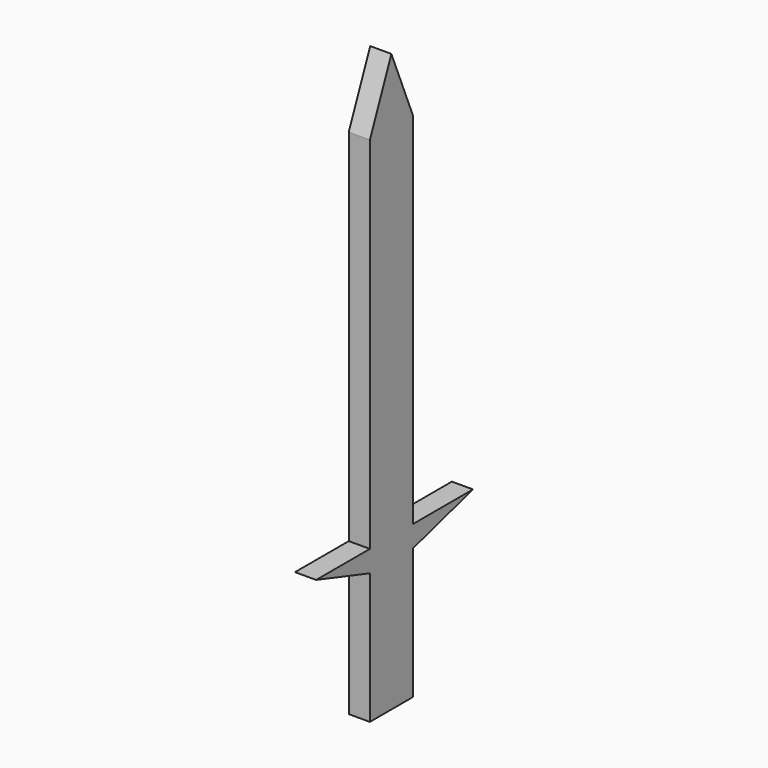
from build123d import *

# Parameters (mm, degrees)
F1_DEPTH    = 2.54
F2_T1_DEPTH = 28.6682991577
F3_DEPTH    = 2.54
F4_DEPTH    = 2.54
F5_T1_DEPTH = 28.6682991577
F6_T1_DEPTH = 28.8815311919


# Not quite as in the source:
# - a fillet or chamfer that OpenCascade refuses, or shapes differently, is made with other operations: its cross-section is extruded or revolved along the edge and cut away or added


with BuildPart() as f1:
    # F0 (on Right) → F1 (new body)
    with BuildSketch(Plane.YZ):
        Polygon((-57.2273433208, -53.503472358), (-49.1374544799, -56.0896545649), (-49.1374544799, -53.503472358), align=None)
        Polygon((-49.1374544799, -53.503472358), (-49.1374544799, -56.0896545649), (-42.6720008254, -56.0896545649), (-42.6720008254, -53.503472358), (-42.6720008254, 0), (-49.1374544799, 0), align=None)
        with BuildLine():
            Line((-42.6720008254, -56.0896545649), (-49.1374544799, -56.0896545649))
            Line((-49.1374544799, -56.0896545649), (-49.1374544799, -67.4042031169))
            ThreePointArc((-49.1374544799, -67.4042031169), (-45.9047276527, -64.1714762896), (-42.6720008254, -67.4042031169))
            Line((-42.6720008254, -67.4042031169), (-42.6720008254, -56.0896545649))
        make_face()
        Polygon((-42.6720008254, -53.503472358), (-42.6720008254, -56.0896545649), (-33.620364964, -53.503472358), align=None)
        with BuildLine():
            ThreePointArc((-42.6720008254, -67.4042031169), (-45.9047276527, -70.6369299442), (-49.1374544799, -67.4042031169))
            Line((-49.1374544799, -67.4042031169), (-49.1374544799, -71.8398466706))
            Line((-49.1374544799, -71.8398466706), (-42.6720008254, -71.8398466706))
            Line((-42.6720008254, -71.8398466706), (-42.6720008254, -67.4042031169))
        make_face()
        with BuildLine():
            ThreePointArc((-42.6720008254, -67.4042031169), (-45.9047276527, -64.1714762896), (-49.1374544799, -67.4042031169))
            ThreePointArc((-49.1374544799, -67.4042031169), (-45.9047276527, -70.6369299442), (-42.6720008254, -67.4042031169))
        make_face()
    extrude(amount=F1_DEPTH)

    # F2: chamfer of 5.08 on 2 edges, made by hand

    # F2_s2 → F2_t1 (cut)
    with BuildSketch(Plane.YZ.offset(-13.0641495789)):
        Polygon((-44.0574544799, 0), (-49.1374544799, -5.08), (-49.1374544799, 0), align=None)
        Polygon((-42.6720008254, -5.08), (-47.7520008254, 0), (-42.6720008254, 0), align=None)
    extrude(amount=F2_T1_DEPTH, mode=Mode.SUBTRACT)

    # F0 (on Right) → F3 (join)
    with BuildSketch(Plane.YZ):
        Polygon((-57.2273433208, -53.503472358), (-49.1374544799, -56.0896545649), (-49.1374544799, -53.503472358), align=None)
        Polygon((-49.1374544799, -53.503472358), (-49.1374544799, -56.0896545649), (-42.6720008254, -56.0896545649), (-42.6720008254, -53.503472358), (-42.6720008254, 0), (-49.1374544799, 0), align=None)
        with BuildLine():
            Line((-42.6720008254, -56.0896545649), (-49.1374544799, -56.0896545649))
            Line((-49.1374544799, -56.0896545649), (-49.1374544799, -67.4042031169))
            ThreePointArc((-49.1374544799, -67.4042031169), (-45.9047276527, -64.1714762896), (-42.6720008254, -67.4042031169))
            Line((-42.6720008254, -67.4042031169), (-42.6720008254, -56.0896545649))
        make_face()
        Polygon((-42.6720008254, -53.503472358), (-42.6720008254, -56.0896545649), (-33.620364964, -53.503472358), align=None)
        with BuildLine():
            ThreePointArc((-42.6720008254, -67.4042031169), (-45.9047276527, -70.6369299442), (-49.1374544799, -67.4042031169))
            Line((-49.1374544799, -67.4042031169), (-49.1374544799, -71.8398466706))
            Line((-49.1374544799, -71.8398466706), (-42.6720008254, -71.8398466706))
            Line((-42.6720008254, -71.8398466706), (-42.6720008254, -67.4042031169))
        make_face()
        with BuildLine():
            ThreePointArc((-42.6720008254, -67.4042031169), (-45.9047276527, -64.1714762896), (-49.1374544799, -67.4042031169))
            ThreePointArc((-49.1374544799, -67.4042031169), (-45.9047276527, -70.6369299442), (-42.6720008254, -67.4042031169))
        make_face()
    extrude(amount=F3_DEPTH)

    # F0 (on Right) → F4 (join)
    with BuildSketch(Plane.YZ):
        Polygon((-57.2273433208, -53.503472358), (-49.1374544799, -56.0896545649), (-49.1374544799, -53.503472358), align=None)
        Polygon((-49.1374544799, -53.503472358), (-49.1374544799, -56.0896545649), (-42.6720008254, -56.0896545649), (-42.6720008254, -53.503472358), (-42.6720008254, 0), (-49.1374544799, 0), align=None)
        with BuildLine():
            Line((-42.6720008254, -56.0896545649), (-49.1374544799, -56.0896545649))
            Line((-49.1374544799, -56.0896545649), (-49.1374544799, -67.4042031169))
            ThreePointArc((-49.1374544799, -67.4042031169), (-45.9047276527, -64.1714762896), (-42.6720008254, -67.4042031169))
            Line((-42.6720008254, -67.4042031169), (-42.6720008254, -56.0896545649))
        make_face()
        Polygon((-42.6720008254, -53.503472358), (-42.6720008254, -56.0896545649), (-33.620364964, -53.503472358), align=None)
        with BuildLine():
            ThreePointArc((-42.6720008254, -67.4042031169), (-45.9047276527, -70.6369299442), (-49.1374544799, -67.4042031169))
            Line((-49.1374544799, -67.4042031169), (-49.1374544799, -71.8398466706))
            Line((-49.1374544799, -71.8398466706), (-42.6720008254, -71.8398466706))
            Line((-42.6720008254, -71.8398466706), (-42.6720008254, -67.4042031169))
        make_face()
        with BuildLine():
            ThreePointArc((-42.6720008254, -67.4042031169), (-45.9047276527, -64.1714762896), (-49.1374544799, -67.4042031169))
            ThreePointArc((-49.1374544799, -67.4042031169), (-45.9047276527, -70.6369299442), (-42.6720008254, -67.4042031169))
        make_face()
    extrude(amount=F4_DEPTH)

    # F5: chamfer of 5.08 on 2 edges, made by hand

    # F5_s2 → F5_t1 (cut)
    with BuildSketch(Plane.YZ.offset(-13.0641495789)):
        Polygon((-49.1374544799, -5.08), (-44.0574544799, 0), (-49.1374544799, 0), align=None)
        Polygon((-42.6720008254, -5.08), (-47.7520008254, 0), (-42.6720008254, 0), align=None)
    extrude(amount=F5_T1_DEPTH, mode=Mode.SUBTRACT)

    # F6: chamfer of 5.08 on 2 edges, made by hand

    # F6_s2 → F6_t1 (cut)
    with BuildSketch(Plane.YZ.offset(-13.170765596)):
        Polygon((-49.1374544799, -10.16), (-45.5453520315, -1.4878975516), (-49.1374544799, -5.08), align=None)
        Polygon((-46.2641032738, -1.4878975516), (-42.6720008254, -10.16), (-42.6720008254, -5.08), align=None)
    extrude(amount=F6_T1_DEPTH, mode=Mode.SUBTRACT)


solid = f1.part
